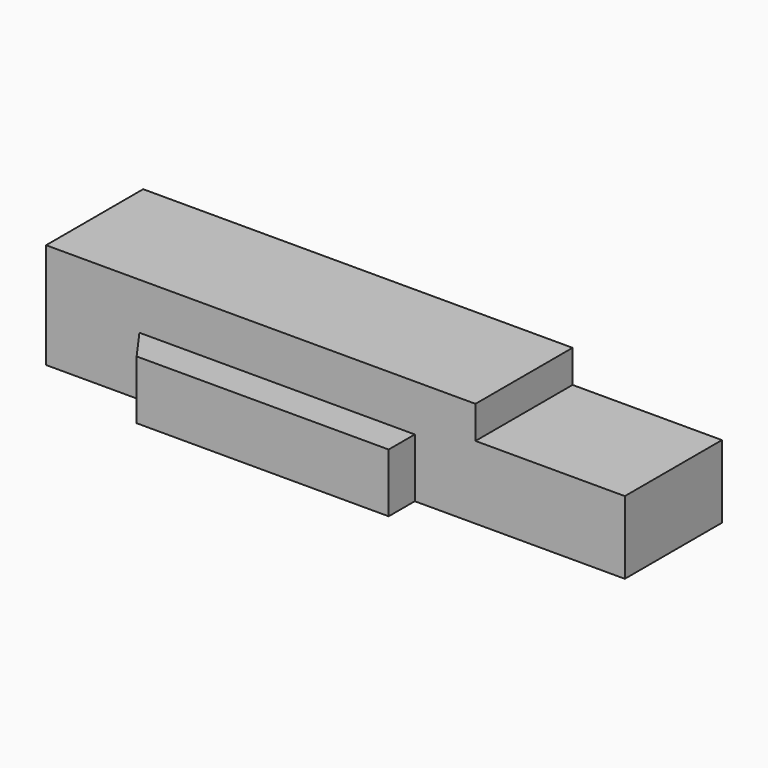
from build123d import *

# Parameters (mm, degrees)
F1_DEPTH      = 12.7
F1_DEPTH_BACK = 12.7
F3_D          = 5.08
F3_DEPTH      = 5.08
F3_TIP        = 1.5261859723
F5_DEPTH      = 92
F4_W          = 8.255
F4_H          = 4.445
F6_DEPTH      = 14.352
F8_W          = 20.32
F8_H          = 4.445
F9_DEPTH      = 9.907
F10_W         = 4.445
F10_H         = 6.35
F11_DEPTH     = 50.166


# Not quite as in the source:
# - an extrude ends at something that could not be found from the text; its depth is read off the source's solid
# - a pattern or mirror of a feature is missing from the dataset's text; its kind, count and spacing are read off the source's solid


with BuildPart() as f1:
    # F0 (on Front) → F1 (new body, two sides)
    with BuildSketch(Plane.XZ) as f1_sk:
        Polygon((-39.37, 14.351), (-39.37, 0), (39.37, 0), (39.37, 9.906), (19.05, 9.906), (19.05, 14.351), align=None)
    extrude(amount=F1_DEPTH)
    extrude(f1_sk.sketch, amount=-F1_DEPTH_BACK)

    # F3
    with Locations(Plane(origin=(-39.37, 0, 0), x_dir=(0, -1, 0), z_dir=(-1, 0, 0))):
        with Locations((0, 10.541)):
            Hole(F3_D / 2, depth=F3_DEPTH)
            with Locations((0, 0, -(F3_DEPTH + F3_TIP / 2))):  # 118° drill point
                Cone(0, F3_D / 2, F3_TIP, mode=Mode.SUBTRACT)

    # F5 (cut, through all): a face of the model
    f5_faces = [f1.faces().sort_by_distance(p)[0] for p in [
        (0, 0, 0),
    ]]
    extrude(f5_faces, amount=F5_DEPTH, mode=Mode.SUBTRACT)

    # F4 (on face) → F6 (cut, through all)
    with BuildSketch(Plane.XY.offset(14.351)):
        Polygon((-39.37, 12.7), (-39.37, 8.255), (-26.67, 8.255), (-23.495, 12.7), align=None)
        with Locations((14.9225, 10.4775)):
            Rectangle(F4_W, F4_H)
    extrude(amount=-F6_DEPTH, mode=Mode.SUBTRACT)

    # F7: F1 across plane


with BuildPart() as f1_1:
    add(f1.part)
    add(f1.part.mirror(Plane.XZ), mode=Mode.INTERSECT)

    # F8 (on face) → F9 (cut, through all)
    with BuildSketch(Plane.XY.offset(9.906)):
        with Locations((29.21, -10.4775)):
            Rectangle(F8_W, F8_H)
        with Locations((29.21, 10.4775)):
            Rectangle(F8_W, F8_H)
    extrude(amount=-F9_DEPTH, mode=Mode.SUBTRACT)

    # F10 (on face) → F11 (cut, through all)
    with BuildSketch(Plane.YZ.offset(10.795)):
        with Locations((10.4775, 11.176)):
            Rectangle(F10_W, F10_H)
    f11 = extrude(amount=-F11_DEPTH, mode=Mode.SUBTRACT)

    # F11_copies: F11 across plane
    add(f11.mirror(Plane(origin=(0, 0, 0), x_dir=(0, 0, -1), z_dir=(0, -1, 0))), mode=Mode.SUBTRACT)


solid = f1_1.part
